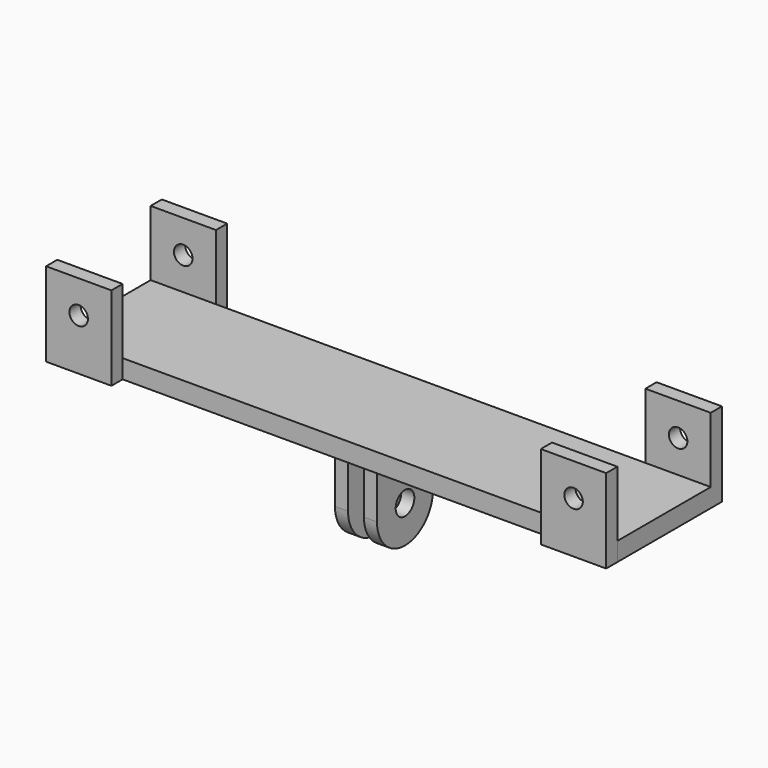
from build123d import *

# Parameters (mm, degrees)
F0_W      = 2.8
F0_H      = 20
F1_DEPTH  = 7.5
F3_R      = 2.5
F4_DEPTH  = 9.001
F5_R      = 7.49999
F5_2_R    = 7.49999
F6_DEPTH  = 12.5
F8_W      = 14
F8_H      = 18
F8_R      = 1.984375
F9_DEPTH  = 3
F11_W     = 14
F11_H     = 18
F11_R     = 1.984375
F12_DEPTH = 3


# Not quite as in the source:
# - a fillet or chamfer is up to 0.001 mm smaller than in the source, because OpenCascade refuses the exact size


with BuildPart() as f1:
    # F0 (on Front) → F1 (new body, symmetric)
    with BuildSketch(Plane.XZ):
        with Locations((-3.1, 0)):
            Rectangle(F0_W, F0_H)
    extrude(amount=F1_DEPTH, both=True)


with BuildPart() as f1b:
    # F0 (on Front) → F1, piece 2 (new body, symmetric)
    with BuildSketch(Plane.XZ):
        with Locations((3.1, 0)):
            Rectangle(F0_W, F0_H)
    extrude(amount=F1_DEPTH, both=True)


with BuildPart() as f4_tool:
    # F3 (on offset) → F4 (new body, through all)
    with BuildSketch(Plane.YZ.offset(4.5)):
        with Locations((0, -2)):
            Circle(F3_R)
    extrude(amount=-F4_DEPTH)


with BuildPart() as f1_1:
    add(f1.part)

    # F4: cut by f4_tool
    add(f4_tool.part, mode=Mode.SUBTRACT)

    # F5#2 (radius 7.5 in the source; OpenCascade refuses exactly that, so slightly less here)
    f5_2_edges = [f1_1.edges().sort_by_distance(p)[0] for p in [
        (-3.1, -7.5, -10),
        (-3.1, 7.5, -10),
    ]]
    fillet(f5_2_edges, radius=F5_2_R)


with BuildPart() as f1b_1:
    add(f1b.part)

    # F4: cut by f4_tool
    add(f4_tool.part, mode=Mode.SUBTRACT)

    # F5 (radius 7.5 in the source; OpenCascade refuses exactly that, so slightly less here)
    f5_edges = [f1b_1.edges().sort_by_distance(p)[0] for p in [
        (3.1, -7.5, -10),
        (3.1, 7.5, -10),
    ]]
    fillet(f5_edges, radius=F5_R)


with BuildPart() as f6:
    # F0 (on Front) → F6 (new body, symmetric)
    with BuildSketch(Plane.XZ):
        Polygon((-1.7, 10), (1.7, 10), (4.5, 10), (60.0000013411, 10), (60.0000013411, 14), (-59.9999986589, 14), (-59.9999986589, 10), (-4.5, 10), align=None)
    extrude(amount=F6_DEPTH, both=True)

    # F8 (on offset) → F9 (join)
    with BuildSketch(Plane.XZ.offset(12.5)):
        with Locations((-52.9999986589, 19)):
            Rectangle(F8_W, F8_H)
        with Locations((-53.0159986589, 20.984375)):
            Circle(F8_R, mode=Mode.SUBTRACT)
        with Locations((52.9999986589, 19)):
            Rectangle(F8_W, F8_H)
        with Locations((53.0159986589, 20.984375)):
            Circle(F8_R, mode=Mode.SUBTRACT)
    extrude(amount=F9_DEPTH)

    # F11 (on offset) → F12 (join)
    with BuildSketch(Plane.XZ.offset(-12.5)):
        with Locations((53.0000013411, 19)):
            Rectangle(F11_W, F11_H)
        with Locations((53.0160013411, 20.984)):
            Circle(F11_R, mode=Mode.SUBTRACT)
        with Locations((-53.0000013411, 19)):
            Rectangle(F11_W, F11_H)
        with Locations((-53.0160013411, 20.984)):
            Circle(F11_R, mode=Mode.SUBTRACT)
    extrude(amount=-F12_DEPTH)


solid = Compound([f1_1.part, f1b_1.part, f6.part])
